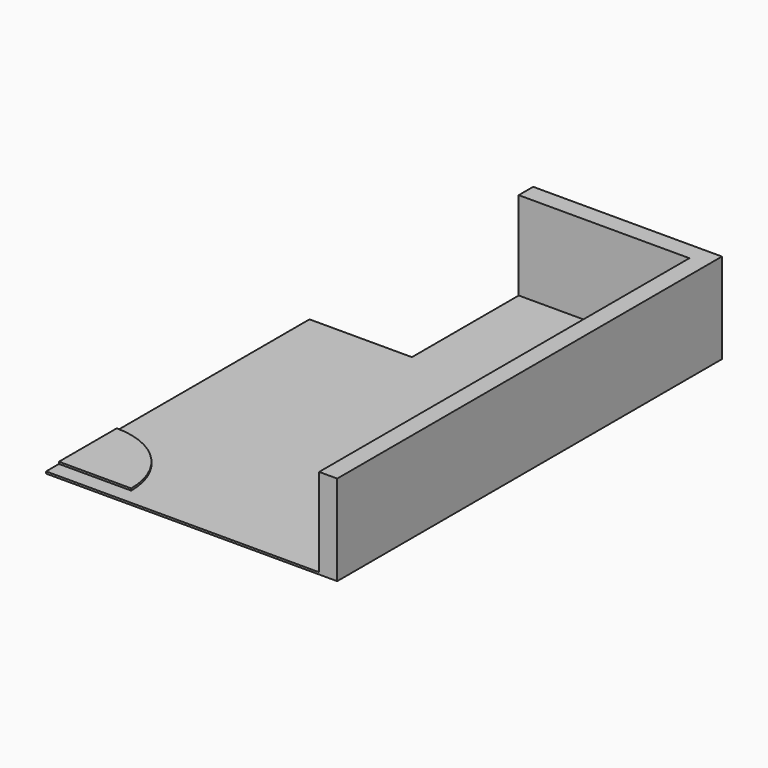
from build123d import *

# Parameters (mm, degrees)
F0_W     = 228.6
F0_H     = 4165.6
F0_W_2   = 279.4
F0_H_2   = 1689.1
F1_DEPTH = 25.4
F2_DEPTH = 25.4
F3_DEPTH = 1117.6


# Not quite as in the source:
# - the program builds the solid bodies; features that only make, move or delete a surface that nothing else refers to are left out


with BuildPart() as f1:
    # F0 (on Top) → F1 (new body)
    with BuildSketch(Plane.XY):
        with BuildLine():
            Line((-3683, 0), (-228.6, 0))
            Line((-228.6, 0), (-228.6, 4165.6))
            Line((-228.6, 4165.6), (-279.4, 4165.6))
            Line((-279.4, 4165.6), (-1041.4, 4165.6))
            Line((-1041.4, 4165.6), (-2108.2, 4165.6))
            Line((-2108.2, 4165.6), (-2387.6, 4165.6))
            Line((-2387.6, 4165.6), (-3683, 4165.6))
            Line((-3683, 4165.6), (-3683, 1117.6))
            ThreePointArc((-3683, 1117.6), (-3036.421559283, 849.778440717), (-2768.6, 203.2))
            Line((-2768.6, 203.2), (-3683, 203.2))
            Line((-3683, 203.2), (-3683, 0))
        make_face()
        with BuildLine():
            Line((-3683, 1117.6), (-3683, 203.2))
            Line((-3683, 203.2), (-2768.6, 203.2))
            ThreePointArc((-2768.6, 203.2), (-3036.421559283, 849.778440717), (-3683, 1117.6))
        make_face()
        with Locations((-114.3, 2082.8)):
            Rectangle(F0_W, F0_H)
        Polygon((-228.6, 4165.6), (0, 4165.6), (0, 6083.3), (-228.6, 6083.3), (-228.6, 5854.7), align=None)
        with BuildLine():
            Line((-279.4, 4165.6), (-228.6, 4165.6))
            Line((-228.6, 4165.6), (-228.6, 5854.7))
            Line((-228.6, 5854.7), (-2108.2, 5854.7))
            Line((-2108.2, 5854.7), (-2108.2, 4165.6))
            Line((-2108.2, 4165.6), (-1041.4, 4165.6))
            Line((-1041.4, 4165.6), (-1041.4, 4927.6))
            ThreePointArc((-1041.4, 4927.6), (-502.5846327359, 4704.4153672641), (-279.4, 4165.6))
        make_face()
        with BuildLine():
            Line((-1041.4, 4165.6), (-279.4, 4165.6))
            ThreePointArc((-279.4, 4165.6), (-502.5846327359, 4704.4153672641), (-1041.4, 4927.6))
            Line((-1041.4, 4927.6), (-1041.4, 4165.6))
        make_face()
        Polygon((-2108.2, 5854.7), (-228.6, 5854.7), (-228.6, 6083.3), (-2387.6, 6083.3), (-2387.6, 5854.7), align=None)
        with Locations((-2247.9, 5010.15)):
            Rectangle(F0_W_2, F0_H_2)
    extrude(amount=-F1_DEPTH)

    # F0 (on Top) → F2 (join)
    with BuildSketch(Plane.XY):
        with BuildLine():
            Line((-3683, 1117.6), (-3683, 203.2))
            Line((-3683, 203.2), (-2768.6, 203.2))
            ThreePointArc((-2768.6, 203.2), (-3036.421559283, 849.778440717), (-3683, 1117.6))
        make_face()
        with BuildLine():
            Line((-1041.4, 4165.6), (-279.4, 4165.6))
            ThreePointArc((-279.4, 4165.6), (-502.5846327359, 4704.4153672641), (-1041.4, 4927.6))
            Line((-1041.4, 4927.6), (-1041.4, 4165.6))
        make_face()
    extrude(amount=F2_DEPTH)

    # F0 (on Top) → F3 (join)
    with BuildSketch(Plane.XY):
        Polygon((-228.6, 4165.6), (0, 4165.6), (0, 6083.3), (-228.6, 6083.3), (-228.6, 5854.7), align=None)
        with Locations((-114.3, 2082.8)):
            Rectangle(F0_W, F0_H)
        Polygon((-2108.2, 5854.7), (-228.6, 5854.7), (-228.6, 6083.3), (-2387.6, 6083.3), (-2387.6, 5854.7), align=None)
    extrude(amount=F3_DEPTH)


solid = f1.part
